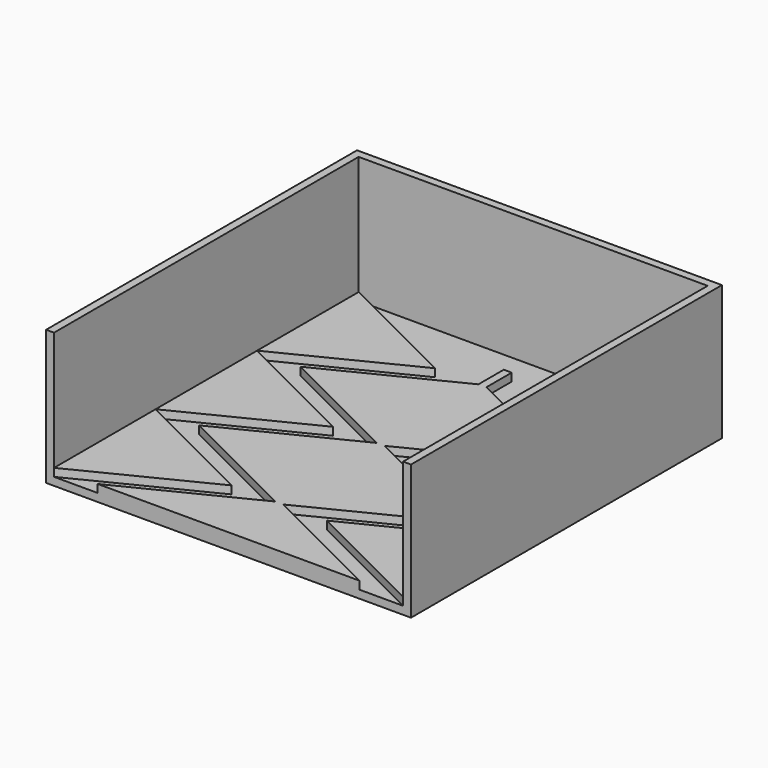
from build123d import *

# Parameters (mm, degrees)
F1_DEPTH = 3.175
F2_DEPTH = 50.8
F3_DEPTH = 3.175


# Not quite as in the source:
# - a length typed as a fraction of an inch, garbled in the dataset ("3 / 203.2 mm" for 3/8 in), is restored


with BuildPart() as f1:
    # F0 (on Top) → F1 (new body)
    with BuildSketch(Plane.XY):
        Polygon((53.975, 25.4), (3.175, 0), (20.638, 0), (71.438, 25.39975), (20.638, 50.7995), (71.438, 76.1995), (20.638, 101.5995), (71.438, 126.9995), (71.438, 139.6995), (74.613, 139.6995), (74.613, 126.9995), (125.412, 101.6), (74.612, 76.2), (125.412, 50.8), (74.612, 25.4), (125.412, 0), (142.875, 0), (92.075, 25.4), (142.875, 50.8), (92.075, 76.2), (142.875, 101.6), (92.075, 127), (142.875, 152.4), (3.175, 152.4), (53.975, 127), (3.175, 101.6), (53.975, 76.2), (3.175, 50.8), align=None)
        Polygon((142.875, 101.6), (142.875, 152.4), (92.075, 127), align=None)
        Polygon((0, 155.575), (0, 0), (3.175, 0), (3.175, 50.8), (3.175, 101.6), (3.175, 152.4), (142.875, 152.4), (142.875, 101.6), (142.875, 50.8), (142.875, 0), (146.05, 0), (146.05, 155.575), align=None)
        Polygon((92.075, 76.2), (142.875, 50.8), (142.875, 101.6), align=None)
        Polygon((92.075, 25.4), (142.875, 0), (142.875, 50.8), align=None)
        Polygon((71.438, 25.39975), (20.638, 0), (125.412, 0), (74.612, 25.4), (125.412, 50.8), (74.612, 76.2), (125.412, 101.6), (74.613, 126.9995), (74.613, 139.6995), (71.438, 139.6995), (71.438, 126.9995), (20.638, 101.5995), (71.438, 76.1995), (20.638, 50.7995), align=None)
        Polygon((3.175, 50.8), (3.175, 0), (53.975, 25.4), align=None)
        Polygon((3.175, 101.6), (3.175, 50.8), (53.975, 76.2), align=None)
        Polygon((3.175, 152.4), (3.175, 101.6), (53.975, 127), align=None)
    extrude(amount=-F1_DEPTH)

    # F0 (on Top) → F2 (join)
    with BuildSketch(Plane.XY):
        Polygon((0, 155.575), (0, 0), (3.175, 0), (3.175, 50.8), (3.175, 101.6), (3.175, 152.4), (142.875, 152.4), (142.875, 101.6), (142.875, 50.8), (142.875, 0), (146.05, 0), (146.05, 155.575), align=None)
    extrude(amount=F2_DEPTH)

    # F0 (on Top) → F3 (join)
    with BuildSketch(Plane.XY):
        Polygon((3.175, 152.4), (3.175, 101.6), (53.975, 127), align=None)
        Polygon((3.175, 101.6), (3.175, 50.8), (53.975, 76.2), align=None)
        Polygon((3.175, 50.8), (3.175, 0), (53.975, 25.4), align=None)
        Polygon((92.075, 25.4), (142.875, 0), (142.875, 50.8), align=None)
        Polygon((92.075, 76.2), (142.875, 50.8), (142.875, 101.6), align=None)
        Polygon((142.875, 101.6), (142.875, 152.4), (92.075, 127), align=None)
        Polygon((71.438, 25.39975), (20.638, 0), (125.412, 0), (74.612, 25.4), (125.412, 50.8), (74.612, 76.2), (125.412, 101.6), (74.613, 126.9995), (74.613, 139.6995), (71.438, 139.6995), (71.438, 126.9995), (20.638, 101.5995), (71.438, 76.1995), (20.638, 50.7995), align=None)
    extrude(amount=F3_DEPTH)


solid = f1.part
